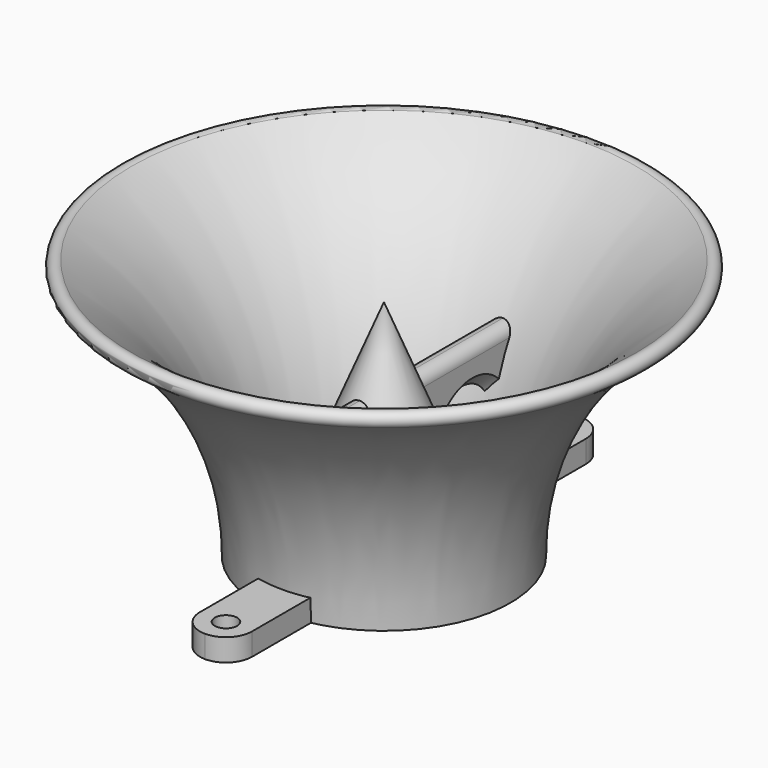
from build123d import *

# Parameters (mm, degrees)
F3_DEPTH   = 3
F4_D       = 3
F4_DEPTH   = 15.81
F4_TIP     = 0.9012909285
F4_2_D     = 3
F4_2_DEPTH = 15.81
F4_2_TIP   = 0.9012909285
F5_W       = 3
F5_H       = 10
F6_DEPTH   = 20.1
F7_R       = 1.49999
F9_DEPTH   = 25
F10_SIZE   = 1.49999
F11_R      = 3.49999
F11_2_R    = 3.49999


# Not quite as in the source:
# - a fillet or chamfer is up to 0.001 mm smaller than in the source, because OpenCascade refuses the exact size


with BuildPart() as f2:
    # F1 (on Front) → F2 (revolve)
    with BuildSketch(Plane.XZ):
        with BuildLine():
            ThreePointArc((-34.9108889941, 33.3187002586), (-21.6749891132, 18.9603630929), (-17, 0))
            Line((-17, 0), (-14.999909446, 0))
            ThreePointArc((-14.999909446, 0), (-19.9334849829, 19.9446773457), (-33.8788173136, 35.0330181488))
            ThreePointArc((-33.8788173136, 35.0330181488), (-35.2790555276, 34.7081760132), (-34.9108889941, 33.3187002586))
        make_face()
    revolve(axis=Axis((0, 0, 33.8666674644), (0, 0, -1)))


with BuildPart() as f2b:
    # F1 (on Front) → F2, piece 2 (revolve)
    with BuildSketch(Plane.XZ):
        Polygon((0, 30), (-12.25, 0), (-9.0095332126, 0), (0, 22.0641629697), align=None)
    revolve(axis=Axis((0, 0, 33.8666674644), (0, 0, -1)))


with BuildPart() as f3:
    # F0 (on Top) → F3 (new body)
    with BuildSketch(Plane.XY):
        with BuildLine():
            Line((3.5, -30), (3.5, -16.6358047596))
            ThreePointArc((3.5, -16.6358047596), (0, -17), (-3.5, -16.6358047596))
            Line((-3.5, -16.6358047596), (-3.5, -30))
            Line((-3.5, -30), (3.5, -30))
        make_face()
    extrude(amount=F3_DEPTH)

    # F4
    with Locations(Plane(origin=(0, 0, 0), x_dir=(1, 0, 0), z_dir=(0, 0, -1))):
        with Locations((0, -30.5), (0, 26.5)):
            Hole(F4_D / 2, depth=F4_DEPTH)
            with Locations((0, 0, -(F4_DEPTH + F4_TIP / 2))):  # 118° drill point
                Cone(0, F4_D / 2, F4_TIP, mode=Mode.SUBTRACT)

    # F11 (radius 3.5 in the source; OpenCascade refuses exactly that, so slightly less here)
    f11_edges = [f3.edges().sort_by_distance(p)[0] for p in [
        (-3.5, -30, 1.5),
        (3.5, -30, 1.5),
    ]]
    fillet(f11_edges, radius=F11_R)


with BuildPart() as f3b:
    # F0 (on Top) → F3, piece 2 (new body)
    with BuildSketch(Plane.XY):
        with BuildLine():
            ThreePointArc((-3.5, 16.6358047596), (0, 17), (3.5, 16.6358047596))
            Line((3.5, 16.6358047596), (3.5, 33))
            Line((3.5, 33), (-3.5, 33))
            Line((-3.5, 33), (-3.5, 16.6358047596))
        make_face()
    extrude(amount=F3_DEPTH)

    # F4#2
    with Locations(Plane(origin=(0, 0, 0), x_dir=(1, 0, 0), z_dir=(0, 0, -1))):
        with Locations((0, -30.5), (0, 26.5)):
            Hole(F4_2_D / 2, depth=F4_2_DEPTH)
            with Locations((0, 0, -(F4_2_DEPTH + F4_2_TIP / 2))):  # 118° drill point
                Cone(0, F4_2_D / 2, F4_2_TIP, mode=Mode.SUBTRACT)

    # F11#2 (radius 3.5 in the source; OpenCascade refuses exactly that, so slightly less here)
    f11_2_edges = [f3b.edges().sort_by_distance(p)[0] for p in [
        (-3.5, 33, 1.5),
        (3.5, 33, 1.5),
    ]]
    fillet(f11_2_edges, radius=F11_2_R)


with BuildPart() as f6:
    # F5 (on Front) → F6 (new body, symmetric)
    with BuildSketch(Plane.XZ):
        with Locations((0, 15)):
            Rectangle(F5_W, F5_H)
    extrude(amount=F6_DEPTH, both=True)

    # F7 (radius 1.5 in the source; OpenCascade refuses exactly that, so slightly less here)
    f7_edges = [f6.edges().sort_by_distance(p)[0] for p in [
        (1.5, 0, 20),
        (-1.5, 0, 20),
    ]]
    fillet(f7_edges, radius=F7_R)

    # F8 (on face) → F9 (cut)
    with BuildSketch(Plane.YZ.offset(1.5)):
        with BuildLine():
            Line((-17.6641202196, 10), (-8.1641202196, 10))
            ThreePointArc((-8.1641202196, 10), (-12.9141202196, 14.75), (-17.6641202196, 10))
        make_face()
        with BuildLine():
            ThreePointArc((-17.6641202196, 10), (-12.9141202196, 5.25), (-8.1641202196, 10))
            Line((-8.1641202196, 10), (-17.6641202196, 10))
        make_face()
        Polygon((-20.1, 10), (-17.6641202196, 10), (-20.1, 16.1745595807), align=None)
        with BuildLine():
            ThreePointArc((17.6641202196, 10), (12.9141202196, 14.75), (8.1641202196, 10))
            Line((8.1641202196, 10), (17.6641202196, 10))
        make_face()
        Polygon((20.1, 16.1745595807), (17.6641202196, 10), (20.1, 10), align=None)
    extrude(amount=-F9_DEPTH, mode=Mode.SUBTRACT)

    # F10 (size 1.5 in the source; OpenCascade refuses exactly that, so slightly less here)
    f10_edges = [f6.edges().sort_by_distance(p)[0] for p in [
        (1.5, -12.91412, 14.75),
        (1.5, 12.91412, 14.75),
        (-1.5, 12.91412, 14.75),
        (-1.5, -12.91412, 14.75),
    ]]
    chamfer(f10_edges, length=F10_SIZE)


solid = Compound([f2.part, f2b.part, f3.part, f3b.part, f6.part])
